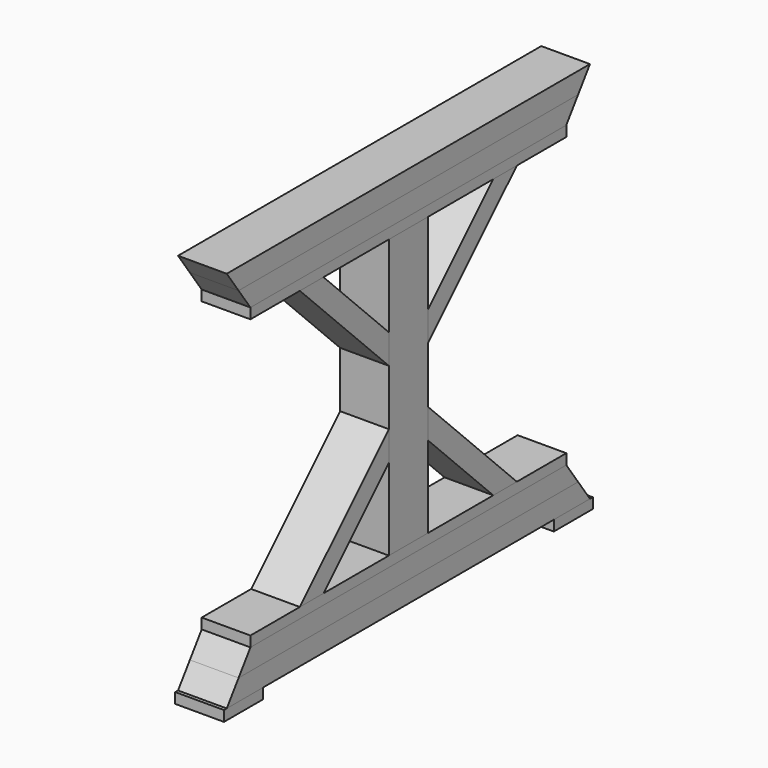
from build123d import *

# Parameters (mm, degrees)
F0_W      = 88.9
F0_H      = 38.1
F1_DEPTH  = 414.3375
F2_W      = 88.9
F2_H      = 38.1
F3_DEPTH  = 414.3375
F5_W      = 88.9
F5_H      = 19.05
F6_DEPTH  = 88.9
F8_W      = 88.9
F8_H      = 19.05
F9_DEPTH  = 360.3625
F11_DEPTH = 88.901
F12_W     = 88.9
F12_H     = 88.9
F13_DEPTH = 508
F17_DEPTH = 88.9


# Not quite as in the source:
# - a feature names something its author has since deleted; it is built from what else it names


with BuildPart() as f1:
    # F0 (on Front) → F1 (new body, symmetric)
    with BuildSketch(Plane.XZ):
        with Locations((44.45, 19.05)):
            Rectangle(F0_W, F0_H)
    extrude(amount=F1_DEPTH, both=True)


with BuildPart() as f3:
    # F2 (on Front) → F3 (new body, symmetric)
    with BuildSketch(Plane.XZ):
        with Locations((44.45, 57.15)):
            Rectangle(F2_W, F2_H)
    extrude(amount=F3_DEPTH, both=True)


with BuildPart() as f6:
    # F5 (on offset) → F6 (new body)
    with BuildSketch(Plane.XZ.offset(420.6875)):
        with Locations((44.45, -9.525)):
            Rectangle(F5_W, F5_H)
    extrude(amount=-F6_DEPTH)


with BuildPart() as f7_1:
    # F7: instance of F6
    add(f6.part.mirror(Plane.XZ))


with BuildPart() as f9:
    # F8 (on Front) → F9 (new body, symmetric)
    with BuildSketch(Plane.XZ):
        with Locations((44.45, 85.725)):
            Rectangle(F8_W, F8_H)
    extrude(amount=F9_DEPTH, both=True)


with BuildPart() as f11_tool:
    # F10 (on face) → F11 (new body, through all)
    with BuildSketch(Plane.YZ.offset(88.9)):
        Polygon((-360.300630331, 76.2), (-414.3375, 76.2), (-414.3375, 38.1), (-387.3190651655, 38.1), align=None)
        Polygon((-387.3190651655, 38.1), (-414.3375, 38.1), (-414.3375, 0), align=None)
        Polygon((414.3375, 76.2), (360.300630331, 76.2), (387.3190651655, 38.1), (414.3375, 38.1), align=None)
        Polygon((414.3375, 38.1), (387.3190651655, 38.1), (414.3375, 0), align=None)
    extrude(amount=-F11_DEPTH)


with BuildPart() as f1_1:
    add(f1.part)

    # F11: cut by f11_tool
    add(f11_tool.part, mode=Mode.SUBTRACT)


with BuildPart() as f3_1:
    add(f3.part)

    # F11: cut by f11_tool
    add(f11_tool.part, mode=Mode.SUBTRACT)


with BuildPart() as f13:
    # F12 (on face) → F13 (new body)
    with BuildSketch(Plane.XY.offset(95.25)):
        with Locations((44.45, 0)):
            Rectangle(F12_W, F12_H)
    extrude(amount=F13_DEPTH)


with BuildPart() as f15_1:
    # F15: instance of F9
    add(f9.part.mirror(Plane.XY.offset(349.25)))


with BuildPart() as f15_2:
    # F15: instance of F3
    add(f3_1.part.mirror(Plane.XY.offset(349.25)))


with BuildPart() as f15_3:
    # F15: instance of F1
    add(f1_1.part.mirror(Plane.XY.offset(349.25)))


with BuildPart() as f17:
    # F16 (on face) → F17 (new body)
    with BuildSketch(Plane(origin=(0, 0, 0), x_dir=(0, -1, 0), z_dir=(-1, 0, 0))):
        Polygon((-247.5565367264, 95.25), (-193.675, 95.25), (-44.45, 244.475), (-44.45, 298.3565367264), align=None)
    extrude(amount=-F17_DEPTH)


with BuildPart() as f18_1:
    # F18: instance of F17
    add(f17.part.mirror(Plane.XZ))


with BuildPart() as f19_1:
    # F19: instance of F17
    add(f17.part.mirror(Plane.XY.offset(349.25)))


with BuildPart() as f19_2:
    # F19: instance of F18_1
    add(f18_1.part.mirror(Plane.XY.offset(349.25)))


solid = Compound([f6.part, f7_1.part, f9.part, f1_1.part, f3_1.part, f13.part, f15_1.part, f15_2.part, f15_3.part, f17.part, f18_1.part, f19_1.part, f19_2.part])
